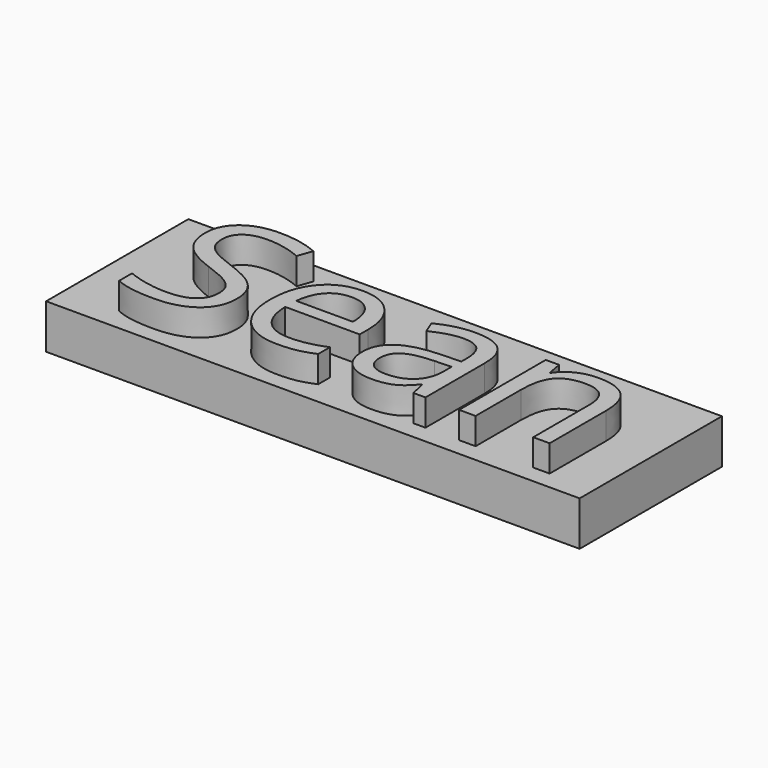
from build123d import *

# Parameters (mm, degrees)
F0_W         = 60
F0_H         = 20
F1_DEPTH     = 5
F2_TEXT_SIZE = 22.7337311736
F3_DEPTH     = 3


# Not quite as in the source:
# - Text() gives the source's letters only with a copy of the font that has no kerning and outlines rounded to 1/6400 em; it was checked with that copy


with BuildPart() as f1:
    # F0 (on Top) → F1 (new body)
    with BuildSketch(Plane.XY):
        Rectangle(F0_W, F0_H)
    extrude(amount=F1_DEPTH)

    # F2 (on face) → F3 (join)
    with BuildSketch(Plane.XY.offset(5)):
        with Locations((-25, -7.968286445)):
            Text('Sean', F2_TEXT_SIZE, font='Open Sans', text_align=(TextAlign.LEFT, TextAlign.BOTTOM))
    extrude(amount=F3_DEPTH)


solid = f1.part
